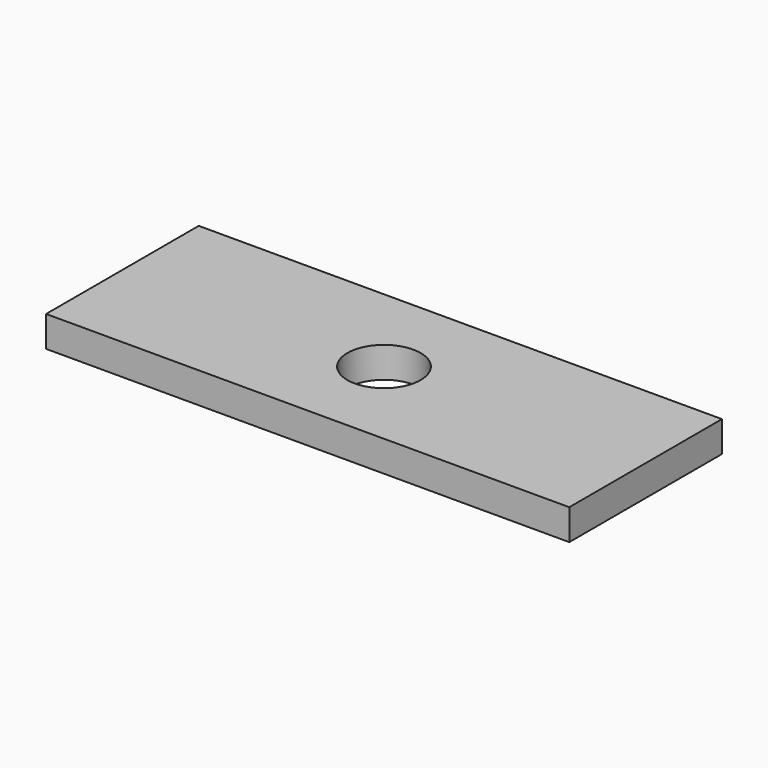
from build123d import *

# Parameters (mm, degrees)
F0_W     = 85
F0_H     = 31
F1_DEPTH = 5
F3_D     = 11.9126


with BuildPart() as f1:
    # F0 (on Top) → F1 (new body)
    with BuildSketch(Plane.XY):
        with Locations((42.5, 15.5)):
            Rectangle(F0_W, F0_H)
    extrude(amount=F1_DEPTH)

    # F3 (through all)
    with Locations(Plane.XY.offset(5)):
        with Locations((42.5, 15.5)):
            Hole(F3_D / 2)


solid = f1.part
